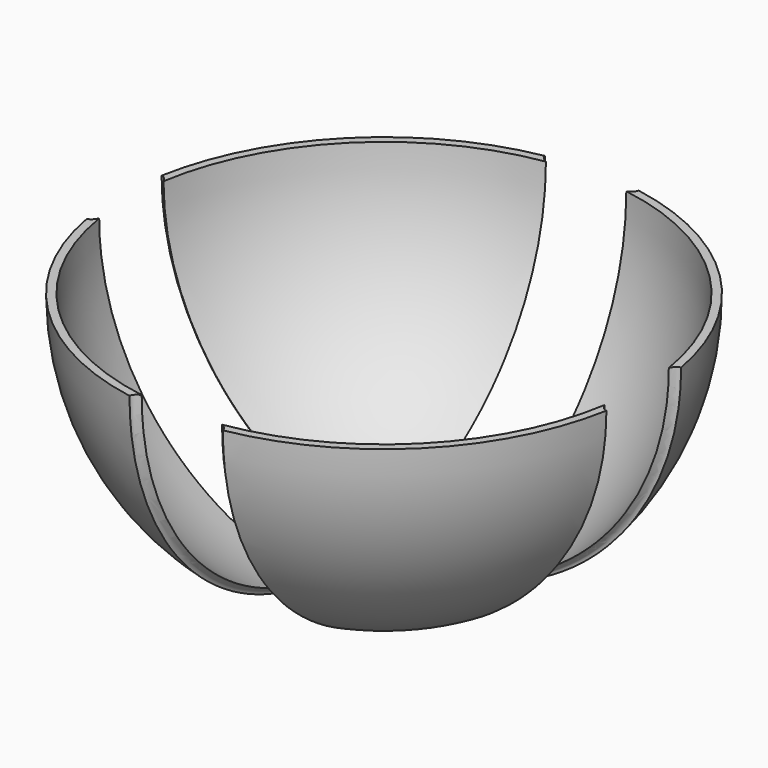
from build123d import *


# Not quite as in the source:
# - the program builds the solid bodies; features that only make, move or delete a surface that nothing else refers to are left out


with BuildPart() as f5:
    # F4 (on Right) → F5 (revolve)
    with BuildSketch(Plane.YZ):
        with BuildLine():
            ThreePointArc((0, -100.0125), (-70.7195169534, -70.7195169534), (-100.0125, 0))
            Line((-100.0125, 0), (-103.1875, 0))
            ThreePointArc((-103.1875, 0), (-72.9645809837, -72.9645809837), (0, -103.1875))
            Line((0, -103.1875), (0, -101.6))
            Line((0, -101.6), (0, -100.0125))
        make_face()
    revolve(axis=Axis((0, 0, -36.2402237952), (0, 0, 1)))

    # F6 (on Top) → F7 (revolve, cut)
    with BuildSketch(Plane.XY):
        with BuildLine():
            add(Edge.make_bspline(
                [(-101.6, 18.25625), (-111.2237072996, 18.25625), (-106.4118536498, -9.128125), (-101.6, -36.5125), (-96.7881463502, -9.128125), (-91.9762927004, 18.25625), (-101.6, 18.25625)],
                knots=[0, 0, 0, 2.0943951024, 2.0943951024, 4.1887902048, 4.1887902048, 6.2831853072, 6.2831853072, 6.2831853072], degree=2, weights=[1, 0.5, 1, 0.5, 1, 0.5, 1]))
        make_face()
    revolve(axis=Axis((0, 24.2510139942, 0), (0, 1, 0)), mode=Mode.SUBTRACT)

    # F8 (on Top) → F9 (revolve, cut)
    with BuildSketch(Plane.XY):
        with BuildLine():
            add(Edge.make_bspline(
                [(18.25625, 101.6), (18.25625, 111.2237072996), (-9.128125, 106.4118536498), (-36.5125, 101.6), (-9.128125, 96.7881463502), (18.25625, 91.9762927004), (18.25625, 101.6)],
                knots=[0, 0, 0, 2.0943951024, 2.0943951024, 4.1887902048, 4.1887902048, 6.2831853072, 6.2831853072, 6.2831853072], degree=2, weights=[1, 0.5, 1, 0.5, 1, 0.5, 1]))
        make_face()
    revolve(axis=Axis((27.766270563, 0, 0), (1, 0, 0)), mode=Mode.SUBTRACT)


solid = f5.part
